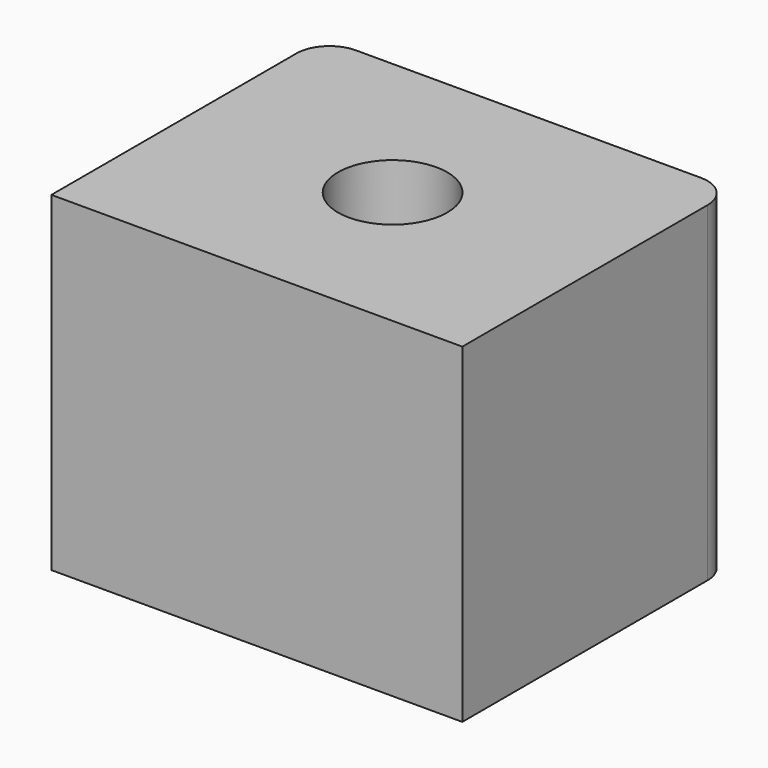
from build123d import *

# Parameters (mm, degrees)
F0_W          = 63.1906017661
F0_H          = 52.1872714162
F0_R          = 8.3960945755
F1_DEPTH      = 25.4
F1_DEPTH_BACK = 25.4
F2_R          = 5.08


# Not quite as in the source:
# - the program builds the solid bodies; features that only make, move or delete a surface that nothing else refers to are left out


with BuildPart() as f1:
    # F0 (on Top) → F1 (new body, two sides)
    with BuildSketch(Plane.XY) as f1_sk:
        Rectangle(F0_W, F0_H)
        Circle(F0_R, mode=Mode.SUBTRACT)
    extrude(amount=F1_DEPTH)
    extrude(f1_sk.sketch, amount=-F1_DEPTH_BACK)

    # F2
    f2_edges = [f1.edges().sort_by_distance(p)[0] for p in [
        (-31.595301, 26.093636, 0),
        (31.595301, 26.093636, 0),
    ]]
    fillet(f2_edges, radius=F2_R)


solid = f1.part
